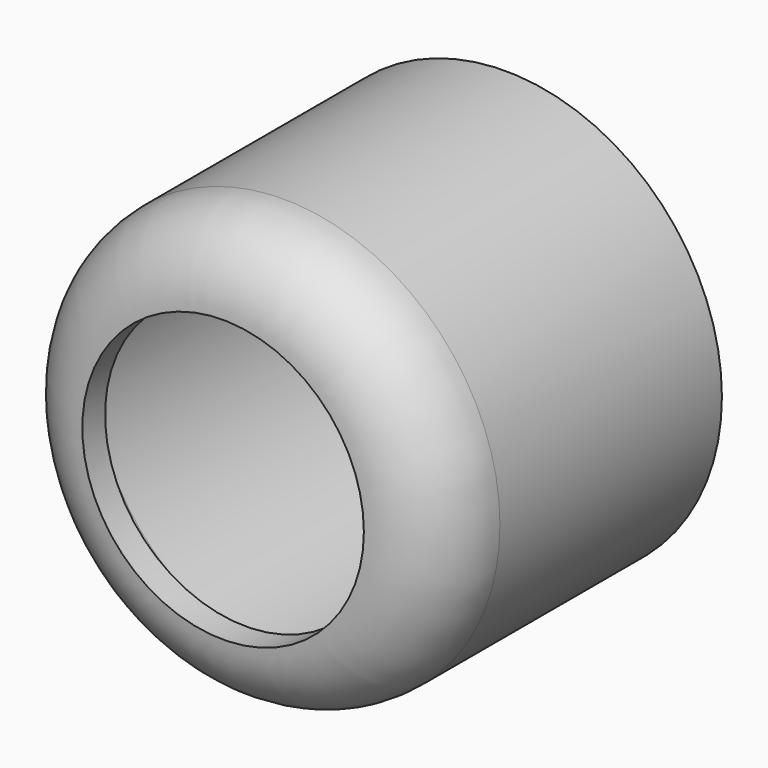
from build123d import *

# Parameters (mm, degrees)
F0_R     = 19.304886182
F1_DEPTH = 31.496
F2_R     = 6.7453126933
F3_T     = -2.54


# Not quite as in the source:
# - a shell that OpenCascade refuses in one call is made with other operations: the cavity is built on its own and cut out


with BuildPart() as f1:
    # F0 (on Front) → F1 (new body)
    with BuildSketch(Plane.XZ):
        with Locations((-28.4389294684, 24.6289279312)):
            Circle(F0_R)
    extrude(amount=F1_DEPTH)

    # F2
    f2_edges = [f1.edges().sort_by_distance(p)[0] for p in [
        (-47.743816, -31.496, 24.628928),
    ]]
    fillet(f2_edges, radius=F2_R)

    # F3: a shell. OpenCascade refuses it in one call, so the cavity is built on its own and cut out:
    # the body offset inwards by the wall thickness, plus a prism from it out through each open face.
    f3_core = offset(f1.part, amount=F3_T, mode=Mode.PRIVATE)
    f3_exits = [f3_core.faces().sort_by_distance(p)[0] for p in [
        (-28.438929, -28.956, 24.628928),
    ]]
    add(f3_core, mode=Mode.SUBTRACT)
    extrude(f3_exits, amount=-F3_T, mode=Mode.SUBTRACT)


solid = f1.part
